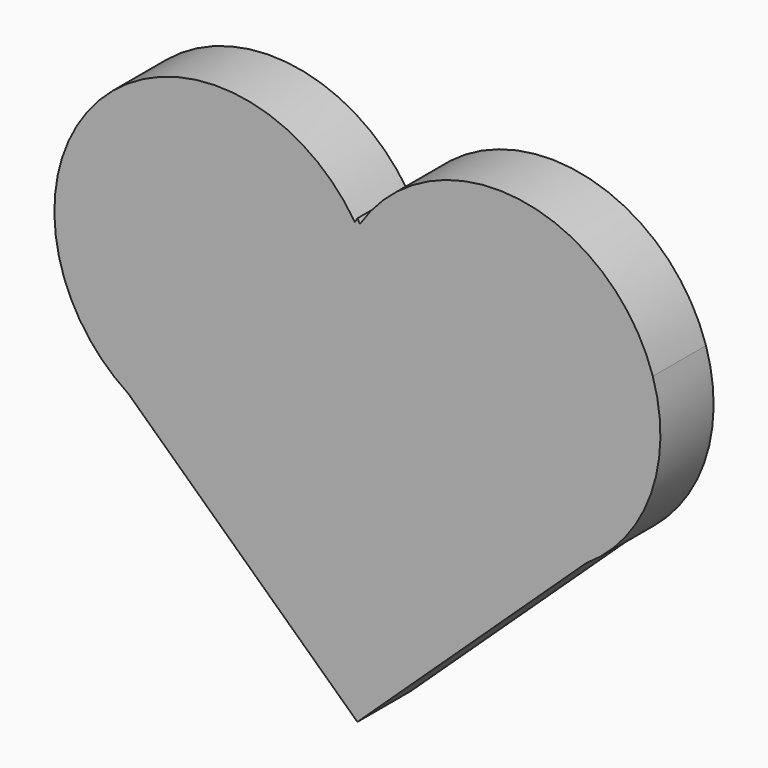
from build123d import *

# Parameters (mm, degrees)
F1_DEPTH = 4.7


# Not quite as in the source:
# - ends of sketch curves that miss each other by under 0.0002 mm in the source are joined


with BuildPart() as f1:
    # F0 (on Front) → F1 (new body)
    with BuildSketch(Plane.XZ):
        with BuildLine():
            ThreePointArc((0, 11.8672233933), (-0.0902475569, 11.7210890642), (-0.178309172, 11.5736271517))
            ThreePointArc((-0.178309172, 11.5736271517), (-11.401199024, 16.7770189855), (-20.8802270777, 8.8286499477))
            ThreePointArc((-20.8802270777, 8.8286499477), (-20.746257812, 1.4589596438), (-16.1770906643, -4.3248967268))
            add(Edge.make_bspline(
                [(-16.1770906643, -4.3248967268), (-10.7847263301, -9.3733878861), (-5.3923627754, -14.4218785382), (7.794e-07, -19.4703691903)],
                knots=[0, 0, 0, 0, 22.160405753, 22.160405753, 22.160405753, 22.160405753], degree=3))
            add(Edge.make_bspline(
                [(16.1770898849, -4.324897234), (10.7847263301, -9.3733878861), (5.3923627754, -14.4218785382), (7.794e-07, -19.4703691903)],
                knots=[0, 0, 0, 0, 22.160405753, 22.160405753, 22.160405753, 22.160405753], degree=3))
            ThreePointArc((16.1770898849, -4.324897234), (20.746257812, 1.4589596438), (20.8802270777, 8.8286499477))
            ThreePointArc((20.8802270777, 8.8286499477), (11.401199024, 16.7770189855), (0.178309172, 11.5736271517))
            ThreePointArc((0.178309172, 11.5736271517), (0.0902475569, 11.7210890642), (0, 11.8672233933))
        make_face()
    extrude(amount=F1_DEPTH)


solid = f1.part
